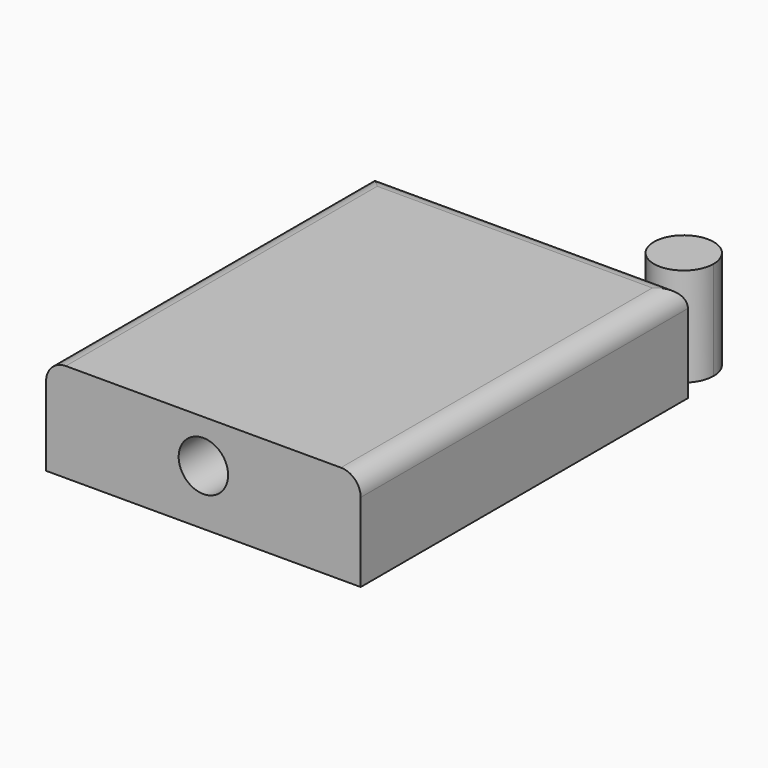
from build123d import *

# Parameters (mm, degrees)
F1_DEPTH    = 25.4
F2_R        = 6.3593196361
F3_DEPTH    = 119.38
F4_T1_DEPTH = 106.3739753604
F4_T3_DEPTH = 130.6661687136


# Not quite as in the source:
# - a fillet or chamfer that OpenCascade refuses, or shapes differently, is made with other operations: its cross-section is extruded or revolved along the edge and cut away or added


with BuildPart() as f1:
    # F0 (on Top) → F1 (new body)
    with BuildSketch(Plane.XY):
        Polygon((40.4869876802, 52.6330843568), (0, 52.6330843568), (-40.4869876802, 52.6330843568), (-40.4869876802, 0), (-40.4869876802, -52.6330843568), (0, -52.6330843568), (40.4869876802, -52.6330843568), (40.4869876802, 0), align=None)
    extrude(amount=F1_DEPTH)

    # F2 (on face) → F3 (cut)
    with BuildSketch(Plane.XZ.offset(52.6330843568)):
        with Locations((0, 14.2668439075)):
            Circle(F2_R)
    extrude(amount=-F3_DEPTH, mode=Mode.SUBTRACT)

    # F4: fillet of radius 5.08 on 3 edges, made by hand

    # F4_s2 → F4_t1 (cut)
    with BuildSketch(Plane.YZ.offset(-53.1869876802)):
        with BuildLine():
            ThreePointArc((52.6330843568, 20.32), (51.1451868052, 23.9121024484), (47.5530843568, 25.4))
            Line((47.5530843568, 25.4), (52.6330843568, 25.4))
            Line((52.6330843568, 25.4), (52.6330843568, 20.32))
        make_face()
    extrude(amount=F4_T1_DEPTH, mode=Mode.SUBTRACT)

    # F4_s4 → F4_t3 (cut)
    with BuildSketch(Plane.XZ.offset(-65.3330843568)):
        with BuildLine():
            ThreePointArc((-35.4069876802, 25.4), (-38.9990901286, 23.9121024484), (-40.4869876802, 20.32))
            Line((-40.4869876802, 20.32), (-40.4869876802, 25.4))
            Line((-40.4869876802, 25.4), (-35.4069876802, 25.4))
        make_face()
        with BuildLine():
            ThreePointArc((40.4869876802, 20.32), (38.9990901286, 23.9121024484), (35.4069876802, 25.4))
            Line((35.4069876802, 25.4), (40.4869876802, 25.4))
            Line((40.4869876802, 25.4), (40.4869876802, 20.32))
        make_face()
    extrude(amount=F4_T3_DEPTH, mode=Mode.SUBTRACT)


with BuildPart() as f1b:
    # F0 (on Top) → F1, piece 2 (new body)
    with BuildSketch(Plane.XY):
        with BuildLine():
            ThreePointArc((32.393171096, 70.9174290403), (24.8444423571, 58.5586318274), (38.4932589397, 63.3993941659))
            ThreePointArc((38.4932589397, 63.3993941659), (36.7764082606, 68.2401565045), (32.393171096, 70.9174290403))
        make_face()
    extrude(amount=F1_DEPTH)


solid = Compound([f1.part, f1b.part])
